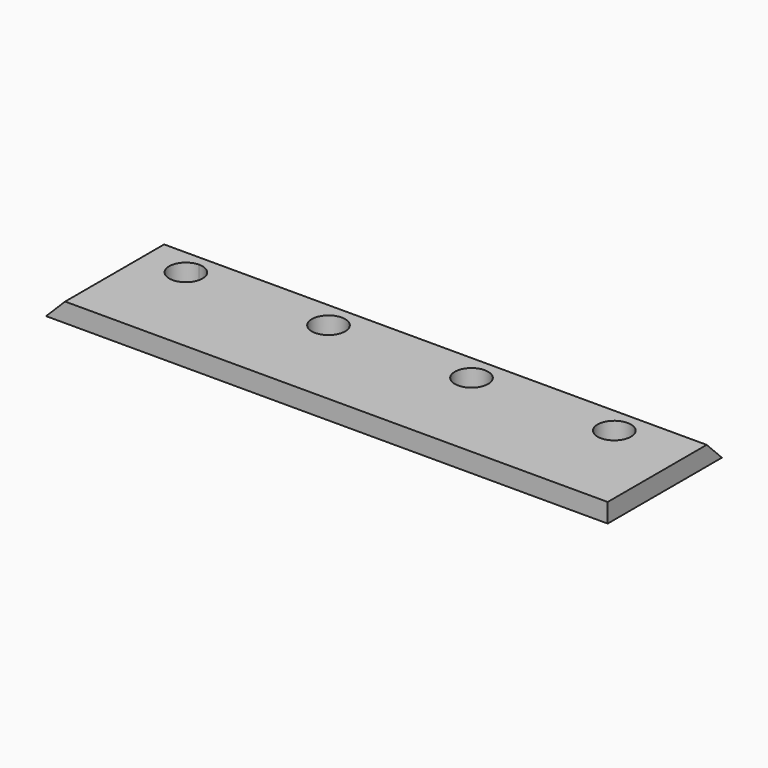
from build123d import *

# Parameters (mm, degrees)
F0_R     = 3.5
F1_DEPTH = 4
F2_SIZE  = 3.99999


# Not quite as in the source:
# - a fillet or chamfer is up to 0.001 mm smaller than in the source, because OpenCascade refuses the exact size


with BuildPart() as f1:
    # F0 (on Top) → F1 (new body)
    with BuildSketch(Plane.XY):
        with BuildLine():
            Line((-60.536339879, 0), (-73.536339879, 0))
            Line((-73.536339879, 0), (-73.536339879, -4))
            Line((-73.536339879, -4), (-73.536339879, -30))
            Line((-73.536339879, -30), (-60.536339879, -30))
            Line((-60.536339879, -30), (-60.536339879, -13.0334984362))
            ThreePointArc((-60.536339879, -13.0334984362), (-64.036339879, -9.5334984362), (-60.536339879, -6.0334984362))
            Line((-60.536339879, -6.0334984362), (-60.536339879, 0))
        make_face()
        with BuildLine():
            Line((44.463660121, 0), (-60.536339879, 0))
            Line((-60.536339879, 0), (-60.536339879, -6.0334984362))
            ThreePointArc((-60.536339879, -6.0334984362), (-58.0614661449, -7.0586247021), (-57.036339879, -9.5334984362))
            ThreePointArc((-57.036339879, -9.5334984362), (-58.0614661449, -12.0083721704), (-60.536339879, -13.0334984362))
            Line((-60.536339879, -13.0334984362), (-60.536339879, -30))
            Line((-60.536339879, -30), (-52.7029968798, -30))
            Line((-52.7029968798, -30), (44.463660121, -30))
            Line((44.463660121, -30), (44.463660121, 0))
        make_face()
        with Locations((-30.536339879, -9.5774214715)):
            Circle(F0_R, mode=Mode.SUBTRACT)
        with Locations((-0.536339879, -9.52560734)):
            Circle(F0_R, mode=Mode.SUBTRACT)
        with Locations((29.463660121, -9.5145422965)):
            Circle(F0_R, mode=Mode.SUBTRACT)
    extrude(amount=F1_DEPTH)

    # F2 (size 4 in the source; OpenCascade refuses exactly that, so slightly less here)
    f2_edges = [f1.edges().sort_by_distance(p)[0] for p in [
        (-73.53634, -15, 4),
        (-14.53634, 0, 4),
    ]]
    chamfer(f2_edges, length=F2_SIZE)


solid = f1.part
